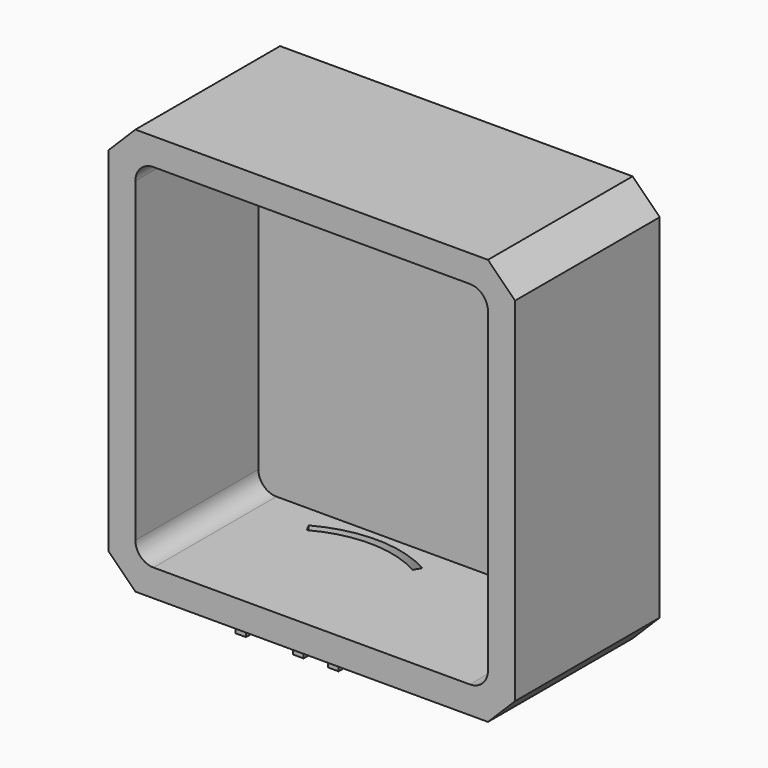
from build123d import *

# Parameters (mm, degrees)
F0_W         = 45
F0_H         = 45
F1_DEPTH     = 20
F2_W         = 39
F2_H         = 39
F3_DEPTH     = 17
F4_R         = 2
F5_SIZE      = 3
F6_TEXT_SIZE = 13.8888888889
F7_DEPTH     = 3
F8_DEPTH     = 3


# Not quite as in the source:
# - Text() gives the source's letters only with a copy of the font that has no kerning and outlines rounded to 1/6400 em; it was checked with that copy


with BuildPart() as f1:
    # F0 (on Front) → F1 (new body)
    with BuildSketch(Plane.XZ):
        Rectangle(F0_W, F0_H)
    extrude(amount=F1_DEPTH)

    # F2 (on face) → F3 (cut, through all)
    with BuildSketch(Plane.XZ.offset(20)):
        Rectangle(F2_W, F2_H)
    extrude(amount=-F3_DEPTH, mode=Mode.SUBTRACT)

    # F4
    f4_edges = [f1.edges().sort_by_distance(p)[0] for p in [
        (19.5, -11.5, 19.5),
        (-19.5, -11.5, 19.5),
        (-19.5, -11.5, -19.5),
        (19.5, -11.5, -19.5),
    ]]
    fillet(f4_edges, radius=F4_R)

    # F5
    f5_edges = [f1.edges().sort_by_distance(p)[0] for p in [
        (22.5, -10, 22.5),
        (-22.5, -10, 22.5),
        (-22.5, -10, -22.5),
        (22.5, -10, -22.5),
    ]]
    chamfer(f5_edges, length=F5_SIZE)

    # F6 (on face) → F7 (join)
    with BuildSketch(Plane(origin=(0, 0, -22.5), x_dir=(1, 0, 0), z_dir=(0, 0, -1))):
        with Locations((-12.8389438614, 6.2624067068)):
            Text('HI', F6_TEXT_SIZE, font='Open Sans', text_align=(TextAlign.LEFT, TextAlign.BOTTOM))
    extrude(amount=F7_DEPTH)

    # F6 (on face) → F8 (cut, through all)
    with BuildSketch(Plane(origin=(0, 0, -22.5), x_dir=(1, 0, 0), z_dir=(0, 0, -1))):
        with BuildLine():
            ThreePointArc((0.2502873249, 6.3671204261), (-5.6262878164, 4.787110164), (-11.5300212055, 6.2624067068))
            Line((-11.5300212055, 6.2624067068), (-11.9604319124, 5.4719976292))
            ThreePointArc((-11.9604319124, 5.4719976292), (-5.6182881432, 3.8871457804), (0.6946806105, 5.584487374))
            Line((0.6946806105, 5.584487374), (0.2502873249, 6.3671204261))
        make_face()
    extrude(amount=-F8_DEPTH, mode=Mode.SUBTRACT)


solid = f1.part
